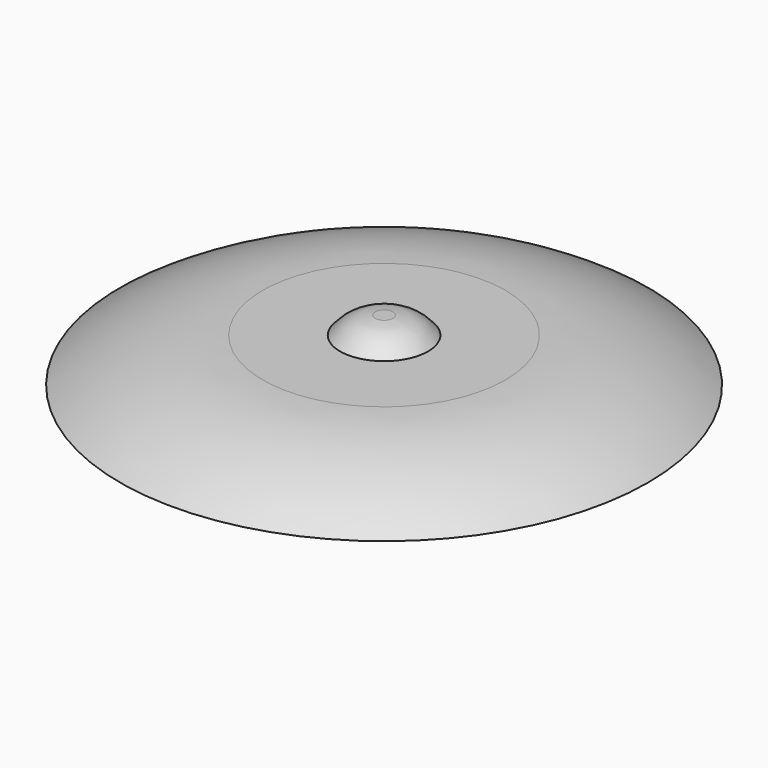
from build123d import *

# Parameters (mm, degrees)
F0_R     = 30
F1_DEPTH = 5
F3_R     = 5
F4_DEPTH = 2
F5_W     = 14.7
F5_H     = 16.5
F6_DEPTH = 1.7


# Not quite as in the source:
# - a fillet or chamfer that OpenCascade refuses, or shapes differently, is made with other operations: its cross-section is extruded or revolved along the edge and cut away or added


with BuildPart() as f1:
    # F0 (on Top) → F1 (new body)
    with BuildSketch(Plane.XY):
        Circle(F0_R)
    extrude(amount=F1_DEPTH)

    # F2: fillet of radius 28.7648476108 on 1 edges, made by hand

    # F2_s1 → F2_t2 (revolve, cut)
    with BuildSketch(Plane.XZ):
        with BuildLine():
            ThreePointArc((30, 0), (22.2736681867, 3.7215915737), (13.7935668295, 5))
            Line((13.7935668295, 5), (30, 5))
            Line((30, 5), (30, 0))
        make_face()
    revolve(axis=Axis((0, 0, 5), (0, 0, 1)), mode=Mode.SUBTRACT)

    # F3 (on face) → F4 (join)
    with BuildSketch(Plane.XY.offset(5)):
        Circle(F3_R)
    extrude(amount=F4_DEPTH)

    # F5 (on face) → F6 (cut)
    with BuildSketch(Plane(origin=(0, 0, 0), x_dir=(1, 0, 0), z_dir=(0, 0, -1))):
        Rectangle(F5_W, F5_H)
    extrude(amount=-F6_DEPTH, mode=Mode.SUBTRACT)

    # F7: fillet of radius 5 on 1 edges, made by hand

    # F7_s1 → F7_t2 (revolve, cut)
    with BuildSketch(Plane.XZ):
        with BuildLine():
            ThreePointArc((5, 5), (3.2360679775, 6.472135955), (1, 7))
            Line((1, 7), (5, 7))
            Line((5, 7), (5, 5))
        make_face()
    revolve(axis=Axis((0, 0, 7), (0, 0, 1)), mode=Mode.SUBTRACT)


solid = f1.part
